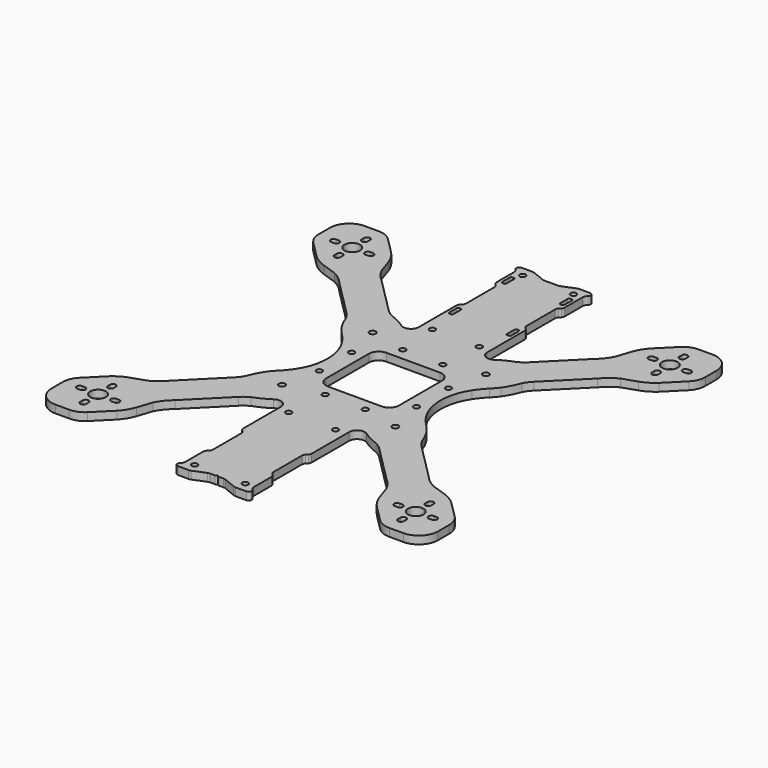
from build123d import *

# Parameters (mm, degrees)
F0_R     = 4
F0_R_2   = 1.5
F0_R_3   = 1.6
F1_DEPTH = 4


# Not quite as in the source:
# - ends of sketch curves that miss each other by under 0.0002 mm in the source are joined


with BuildPart() as f1:
    # F0 (on Top) → F1 (new body)
    with BuildSketch(Plane.XY):
        with BuildLine():
            ThreePointArc((-68.7198979633, -19.2310683136), (-69.2667474289, -19.0706292261), (-69.8340699923, -19.0164983863))
            Line((-69.8340699923, -19.0164983863), (-75.2563229923, -19.0164983863))
            ThreePointArc((-75.2563229923, -19.0164983863), (-76.6575815321, -19.9812652551), (-76.2563229867, -21.63453238))
            ThreePointArc((-76.2563229867, -21.63453238), (-75.5177102079, -22.645855508), (-75.2563229923, -23.8706003863))
            Line((-75.2563229923, -23.8706003863), (-75.2563229923, -35.1880713863))
            ThreePointArc((-75.2563229923, -35.1880713863), (-75.1040821926, -35.9534379244), (-74.6705370547, -36.6022844487))
            Line((-74.6705370547, -36.6022844487), (-73.8421089923, -37.4307123863))
            ThreePointArc((-73.8421089923, -37.4307123863), (-73.408563792, -38.0795588482), (-73.2563229923, -38.8449253863))
            Line((-73.2563229923, -38.8449253863), (-73.2563229923, -57.1880713863))
            ThreePointArc((-73.2563229923, -57.1880713863), (-73.408563792, -57.9534379244), (-73.8421089299, -58.6022844487))
            Line((-73.8421089299, -58.6022844487), (-74.6705369923, -59.4307123863))
            ThreePointArc((-74.6705369923, -59.4307123863), (-75.1040821926, -60.0795588482), (-75.2563229923, -60.8449253863))
            Line((-75.2563229923, -60.8449253863), (-75.2563229923, -84.8364823863))
            ThreePointArc((-75.2563229923, -84.8364823863), (-77.3940816238, -88.3765469458), (-81.5223515351, -88.1327097212))
            ThreePointArc((-81.5223515351, -88.1327097212), (-85.5001057777, -85.7657105269), (-89.7529047165, -83.9384406075))
            ThreePointArc((-89.7529047165, -83.9384406075), (-91.8824323761, -82.6525966161), (-93.7563230573, -81.0164984487))
            Line((-93.7563230573, -81.0164984487), (-111.8499919923, -62.9020143863))
            ThreePointArc((-111.8499919923, -62.9020143863), (-115.0500186095, -59.6637600428), (-117.5068461048, -55.8309464428))
            Line((-117.5068461048, -55.8309464428), (-119.9817199923, -48.4063253863))
            ThreePointArc((-119.9817199923, -48.4063253863), (-121.7314401326, -44.6478315667), (-124.2243601054, -41.3352574916))
            Line((-124.2243601054, -41.3352574916), (-132.7096419923, -32.8499763863))
            ThreePointArc((-132.7096419923, -32.8499763863), (-135.9638712469, -30.7325010032), (-139.7807099968, -30.0215490151))
            Line((-139.7807099968, -30.0215490151), (-146.8517769923, -30.0215493863))
            ThreePointArc((-146.8517769923, -30.0215493863), (-153.8517770371, -32.9210443415), (-156.7512719923, -39.9210443863))
            Line((-156.7512719923, -39.9210443863), (-156.7512719923, -46.9921113863))
            ThreePointArc((-156.7512719923, -46.9921113863), (-156.0403203754, -50.8089501317), (-153.9228453387, -54.0631797243))
            Line((-153.9228453387, -54.0631797243), (-145.4375639923, -62.5484613863))
            ThreePointArc((-145.4375639923, -62.5484613863), (-142.1249898119, -65.0413812461), (-138.3664962297, -66.7911020771))
            Line((-138.3664962297, -66.7911020771), (-130.9418749923, -69.2659753863))
            ThreePointArc((-130.9418749923, -69.2659753863), (-127.1090613358, -71.7228027691), (-123.870807081, -74.922829459))
            Line((-123.870807081, -74.922829459), (-105.8395839923, -92.9540523863))
            ThreePointArc((-105.8395839923, -92.9540523863), (-104.1591231129, -94.8555234649), (-102.8343796027, -97.0199161923))
            ThreePointArc((-102.8343796027, -97.0199161923), (-101.008160191, -101.2706562812), (-98.6427303315, -105.2466606194))
            ThreePointArc((-98.6427303315, -105.2466606194), (-97.1356962685, -107.0614279538), (-95.5198284171, -108.7800038111))
            ThreePointArc((-95.5198284171, -108.7800038111), (-93.1084062482, -111.4552655604), (-90.9867028572, -114.3656532981))
            ThreePointArc((-90.9867028572, -114.3656532981), (-86.6660489281, -129.0164983863), (-90.9867028572, -143.6673434744))
            ThreePointArc((-90.9867028572, -143.6673434744), (-93.1084062482, -146.5777312121), (-95.5198288752, -149.2529925034))
            ThreePointArc((-95.5198288752, -149.2529925034), (-97.1356962685, -150.9715688188), (-98.6427295666, -152.7863367182))
            ThreePointArc((-98.6427295666, -152.7863367182), (-101.008160191, -156.7623404914), (-102.8343807712, -161.0130801105))
            ThreePointArc((-102.8343807712, -161.0130801105), (-104.1591231129, -163.1774733076), (-105.8395836562, -165.0789447401))
            Line((-105.8395836562, -165.0789447401), (-123.8708069923, -183.1101673863))
            ThreePointArc((-123.8708069923, -183.1101673863), (-127.1090613358, -186.3101940035), (-130.9418749358, -188.7670214988))
            Line((-130.9418749358, -188.7670214988), (-138.3664959923, -191.2418953863))
            ThreePointArc((-138.3664959923, -191.2418953863), (-142.1249898119, -192.9916155265), (-145.437563887, -195.4845354993))
            Line((-145.437563887, -195.4845354993), (-153.9228449923, -203.9698173863))
            ThreePointArc((-153.9228449923, -203.9698173863), (-156.0403203754, -207.2240466409), (-156.7512723635, -211.0408853908))
            Line((-156.7512723635, -211.0408853908), (-156.7512719923, -218.1119523863))
            ThreePointArc((-156.7512719923, -218.1119523863), (-153.8517770371, -225.1119524311), (-146.8517769923, -228.0114473863))
            Line((-146.8517769923, -228.0114473863), (-139.7807099923, -228.0114473863))
            ThreePointArc((-139.7807099923, -228.0114473863), (-135.9638712469, -227.3004957694), (-132.7096416543, -225.1830207326))
            Line((-132.7096416543, -225.1830207326), (-124.2243599923, -216.6977393863))
            ThreePointArc((-124.2243599923, -216.6977393863), (-121.7314401326, -213.3851652059), (-119.9817193015, -209.6266716237))
            Line((-119.9817193015, -209.6266716237), (-117.5068459923, -202.2020503863))
            ThreePointArc((-117.5068459923, -202.2020503863), (-115.0500186095, -198.3692367297), (-111.8499919196, -195.130982475))
            Line((-111.8499919196, -195.130982475), (-93.7563229923, -177.0164983863))
            ThreePointArc((-93.7563229923, -177.0164983863), (-91.8824323761, -175.3804001564), (-89.7529048375, -174.0945557019))
            ThreePointArc((-89.7529048375, -174.0945557019), (-85.5001057777, -172.2672862456), (-81.5223513734, -169.9002872866))
            ThreePointArc((-81.5223513734, -169.9002872866), (-77.3940816238, -169.6564498268), (-75.2563229923, -173.1965143863))
            Line((-75.2563229923, -173.1965143863), (-75.2563229923, -197.1880713863))
            ThreePointArc((-75.2563229923, -197.1880713863), (-75.1040821926, -197.9534379244), (-74.6705370547, -198.6022844487))
            Line((-74.6705370547, -198.6022844487), (-73.8421089923, -199.4307123863))
            ThreePointArc((-73.8421089923, -199.4307123863), (-73.408563792, -200.0795588482), (-73.2563229923, -200.8449253863))
            Line((-73.2563229923, -200.8449253863), (-73.2563229923, -219.1880713863))
            ThreePointArc((-73.2563229923, -219.1880713863), (-73.408563792, -219.9534379244), (-73.8421089299, -220.6022844487))
            Line((-73.8421089299, -220.6022844487), (-74.6705369923, -221.4307123863))
            ThreePointArc((-74.6705369923, -221.4307123863), (-75.1040821926, -222.0795588482), (-75.2563229923, -222.8449253863))
            Line((-75.2563229923, -222.8449253863), (-75.2563229923, -234.1623963863))
            ThreePointArc((-75.2563229923, -234.1623963863), (-75.5177102079, -235.3871412645), (-76.2563230035, -236.3984643738))
            ThreePointArc((-76.2563230035, -236.3984643738), (-76.6575815321, -238.0517315174), (-75.2563229923, -239.0164983863))
            Line((-75.2563229923, -239.0164983863), (-69.8340699923, -239.0164983863))
            ThreePointArc((-69.8340699923, -239.0164983863), (-69.2667474289, -238.9623675465), (-68.7198979633, -238.8019284589))
            Line((-68.7198979633, -238.8019284589), (-62.2927479923, -236.2310683863))
            ThreePointArc((-62.2927479923, -236.2310683863), (-61.7458985558, -236.0706292261), (-61.1785759923, -236.0164983863))
            Line((-61.1785759923, -236.0164983863), (-58.7563229923, -236.0164983863))
            ThreePointArc((-58.7563229923, -236.0164983863), (-58.0492162111, -235.7236051675), (-57.7563229923, -235.0164983863))
            ThreePointArc((-57.7563229923, -235.0164983863), (-57.4634297735, -235.7236051675), (-56.7563229923, -236.0164983863))
            Line((-56.7563229923, -236.0164983863), (-54.3340699923, -236.0164983863))
            ThreePointArc((-54.3340699923, -236.0164983863), (-53.7667474289, -236.0706292261), (-53.2198979633, -236.2310683136))
            Line((-53.2198979633, -236.2310683136), (-46.7927479923, -238.8019283863))
            ThreePointArc((-46.7927479923, -238.8019283863), (-46.2458985558, -238.9623675465), (-45.6785759923, -239.0164983863))
            Line((-45.6785759923, -239.0164983863), (-40.2563229923, -239.0164983863))
            ThreePointArc((-40.2563229923, -239.0164983863), (-38.8550644525, -238.0517315174), (-39.2563229979, -236.3984643925))
            ThreePointArc((-39.2563229979, -236.3984643925), (-39.9949357768, -235.3871412645), (-40.2563229923, -234.1623963863))
            Line((-40.2563229923, -234.1623963863), (-40.2563229923, -222.8449253863))
            ThreePointArc((-40.2563229923, -222.8449253863), (-40.408563792, -222.0795588482), (-40.8421089299, -221.4307123239))
            Line((-40.8421089299, -221.4307123239), (-41.6705369923, -220.6022843863))
            ThreePointArc((-41.6705369923, -220.6022843863), (-42.1040821926, -219.9534379244), (-42.2563229923, -219.1880713863))
            Line((-42.2563229923, -219.1880713863), (-42.2563229923, -200.8449253863))
            ThreePointArc((-42.2563229923, -200.8449253863), (-42.1040821926, -200.0795588482), (-41.6705370547, -199.4307123239))
            Line((-41.6705370547, -199.4307123239), (-40.8421089923, -198.6022843863))
            ThreePointArc((-40.8421089923, -198.6022843863), (-40.408563792, -197.9534379244), (-40.2563229923, -197.1880713863))
            Line((-40.2563229923, -197.1880713863), (-40.2563229923, -173.1965143863))
            ThreePointArc((-40.2563229923, -173.1965143863), (-38.1185643608, -169.6564498268), (-33.9902944496, -169.9002870514))
            ThreePointArc((-33.9902944496, -169.9002870514), (-30.012540207, -172.2672862456), (-25.7597412681, -174.0945561651))
            ThreePointArc((-25.7597412681, -174.0945561651), (-23.6302136086, -175.3804001564), (-21.7563229274, -177.0164983238))
            Line((-21.7563229274, -177.0164983238), (-3.6626539923, -195.1309823863))
            ThreePointArc((-3.6626539923, -195.1309823863), (-0.4626273751, -198.3692367297), (1.9942001202, -202.2020503298))
            Line((1.9942001202, -202.2020503298), (4.4690740077, -209.6266713863))
            ThreePointArc((4.4690740077, -209.6266713863), (6.2187941479, -213.3851652059), (8.7117141207, -216.697739281))
            Line((8.7117141207, -216.697739281), (17.1969960077, -225.1830203863))
            ThreePointArc((17.1969960077, -225.1830203863), (20.4512252623, -227.3004957694), (24.2680640122, -228.0114477575))
            Line((24.2680640122, -228.0114477575), (31.3391310077, -228.0114473863))
            ThreePointArc((31.3391310077, -228.0114473863), (38.3391310525, -225.1119524311), (41.2386260077, -218.1119523863))
            Line((41.2386260077, -218.1119523863), (41.2386260077, -211.0408853863))
            ThreePointArc((41.2386260077, -211.0408853863), (40.5276743908, -207.2240466409), (38.410199354, -203.9698170483))
            Line((38.410199354, -203.9698170483), (29.9249180077, -195.4845353863))
            ThreePointArc((29.9249180077, -195.4845353863), (26.6123438273, -192.9916155265), (22.8538502451, -191.2418946955))
            Line((22.8538502451, -191.2418946955), (15.4292290077, -188.7670213863))
            ThreePointArc((15.4292290077, -188.7670213863), (11.5964153511, -186.3101940035), (8.3581610964, -183.1101673136))
            Line((8.3581610964, -183.1101673136), (-9.6730619923, -165.0789443863))
            ThreePointArc((-9.6730619923, -165.0789443863), (-11.3535228717, -163.1774733076), (-12.678266382, -161.0130805803))
            ThreePointArc((-12.678266382, -161.0130805803), (-14.5044857937, -156.7623404914), (-16.8699156531, -152.7863361531))
            ThreePointArc((-16.8699156531, -152.7863361531), (-18.3769497162, -150.9715688188), (-19.9928175675, -149.2529929615))
            ThreePointArc((-19.9928175675, -149.2529929615), (-22.4042397365, -146.5777312121), (-24.5259431274, -143.6673434744))
            ThreePointArc((-24.5259431274, -143.6673434744), (-28.8465970565, -129.0164983863), (-24.5259431274, -114.3656532981))
            ThreePointArc((-24.5259431274, -114.3656532981), (-22.4042397365, -111.4552655604), (-19.9928171095, -108.7800042691))
            ThreePointArc((-19.9928171095, -108.7800042691), (-18.3769497162, -107.0614279538), (-16.869916418, -105.2466600544))
            ThreePointArc((-16.869916418, -105.2466600544), (-14.5044857937, -101.2706562812), (-12.6782652135, -97.0199166621))
            ThreePointArc((-12.6782652135, -97.0199166621), (-11.3535228717, -94.8555234649), (-9.6730623284, -92.9540520325))
            Line((-9.6730623284, -92.9540520325), (8.3581610077, -74.9228293863))
            ThreePointArc((8.3581610077, -74.9228293863), (11.5964153511, -71.7228027691), (15.4292289512, -69.2659752738))
            Line((15.4292289512, -69.2659752738), (22.8538500077, -66.7911013863))
            ThreePointArc((22.8538500077, -66.7911013863), (26.6123438273, -65.0413812461), (29.9249179024, -62.5484612732))
            Line((29.9249179024, -62.5484612732), (38.4101990077, -54.0631793863))
            ThreePointArc((38.4101990077, -54.0631793863), (40.5276743908, -50.8089501317), (41.2386263789, -46.9921113818))
            Line((41.2386263789, -46.9921113818), (41.2386260077, -39.9210443863))
            ThreePointArc((41.2386260077, -39.9210443863), (38.3391310525, -32.9210443415), (31.3391310077, -30.0215493863))
            Line((31.3391310077, -30.0215493863), (24.2680640077, -30.0215493863))
            ThreePointArc((24.2680640077, -30.0215493863), (20.4512252623, -30.7325010032), (17.1969956697, -32.8499760399))
            Line((17.1969956697, -32.8499760399), (8.7117140077, -41.3352573863))
            ThreePointArc((8.7117140077, -41.3352573863), (6.2187941479, -44.6478315667), (4.4690733169, -48.4063251489))
            Line((4.4690733169, -48.4063251489), (1.9942000077, -55.8309463863))
            ThreePointArc((1.9942000077, -55.8309463863), (-0.4626273751, -59.6637600428), (-3.662654065, -62.9020142976))
            Line((-3.662654065, -62.9020142976), (-21.7563229923, -81.0164983863))
            ThreePointArc((-21.7563229923, -81.0164983863), (-23.6302136086, -82.6525966161), (-25.7597411471, -83.9384410707))
            ThreePointArc((-25.7597411471, -83.9384410707), (-30.012540207, -85.7657105269), (-33.9902946113, -88.1327094859))
            ThreePointArc((-33.9902946113, -88.1327094859), (-38.1185643608, -88.3765469458), (-40.2563229923, -84.8364823863))
            Line((-40.2563229923, -84.8364823863), (-40.2563229923, -60.8449253863))
            ThreePointArc((-40.2563229923, -60.8449253863), (-40.408563792, -60.0795588482), (-40.8421089299, -59.4307123239))
            Line((-40.8421089299, -59.4307123239), (-41.6705369923, -58.6022843863))
            ThreePointArc((-41.6705369923, -58.6022843863), (-42.1040821926, -57.9534379244), (-42.2563229923, -57.1880713863))
            Line((-42.2563229923, -57.1880713863), (-42.2563229923, -38.8449253863))
            ThreePointArc((-42.2563229923, -38.8449253863), (-42.1040821926, -38.0795588482), (-41.6705370547, -37.4307123239))
            Line((-41.6705370547, -37.4307123239), (-40.8421089923, -36.6022843863))
            ThreePointArc((-40.8421089923, -36.6022843863), (-40.408563792, -35.9534379244), (-40.2563229923, -35.1880713863))
            Line((-40.2563229923, -35.1880713863), (-40.2563229923, -23.8706003863))
            ThreePointArc((-40.2563229923, -23.8706003863), (-39.9949357768, -22.645855508), (-39.2563229811, -21.6345323988))
            ThreePointArc((-39.2563229811, -21.6345323988), (-38.8550644525, -19.9812652551), (-40.2563229923, -19.0164983863))
            Line((-40.2563229923, -19.0164983863), (-45.6785759923, -19.0164983863))
            ThreePointArc((-45.6785759923, -19.0164983863), (-46.2458985558, -19.0706292261), (-46.7927480214, -19.2310683136))
            Line((-46.7927480214, -19.2310683136), (-53.2198979923, -21.8019283863))
            ThreePointArc((-53.2198979923, -21.8019283863), (-53.7667474289, -21.9623675465), (-54.3340699923, -22.0164983863))
            Line((-54.3340699923, -22.0164983863), (-56.7563229923, -22.0164983863))
            Line((-56.7563229923, -22.0164983863), (-58.7563229923, -22.0164983863))
            Line((-58.7563229923, -22.0164983863), (-61.1785759923, -22.0164983863))
            ThreePointArc((-61.1785759923, -22.0164983863), (-61.7458985558, -21.9623675465), (-62.2927480214, -21.8019284589))
            Line((-62.2927480214, -21.8019284589), (-68.7198979633, -19.2310683136))
        make_face()
        with BuildLine():
            Line((-137.5736029923, -218.3337783863), (-137.5736029923, -219.8337783863))
            ThreePointArc((-137.5736029923, -219.8337783863), (-139.0736029923, -221.3337783863), (-140.5736029923, -219.8337783863))
            Line((-140.5736029923, -219.8337783863), (-140.5736029923, -218.3337783863))
            ThreePointArc((-140.5736029923, -218.3337783863), (-139.0736029923, -216.8337783863), (-137.5736029923, -218.3337783863))
        make_face(mode=Mode.SUBTRACT)
        with BuildLine():
            Line((-147.0736029923, -211.8337783863), (-148.5736029923, -211.8337783863))
            ThreePointArc((-148.5736029923, -211.8337783863), (-150.0736029923, -210.3337783863), (-148.5736029923, -208.8337783863))
            Line((-148.5736029923, -208.8337783863), (-147.0736029923, -208.8337783863))
            ThreePointArc((-147.0736029923, -208.8337783863), (-145.5736029923, -210.3337783863), (-147.0736029923, -211.8337783863))
        make_face(mode=Mode.SUBTRACT)
        with Locations((-139.0736029923, -210.3337783863)):
            Circle(F0_R, mode=Mode.SUBTRACT)
        with BuildLine():
            Line((-137.5736029923, -200.8337783863), (-137.5736029923, -202.3337783863))
            ThreePointArc((-137.5736029923, -202.3337783863), (-139.0736029923, -203.8337783863), (-140.5736029923, -202.3337783863))
            Line((-140.5736029923, -202.3337783863), (-140.5736029923, -200.8337783863))
            ThreePointArc((-140.5736029923, -200.8337783863), (-139.0736029923, -199.3337783863), (-137.5736029923, -200.8337783863))
        make_face(mode=Mode.SUBTRACT)
        with BuildLine():
            ThreePointArc((-129.5736029923, -208.8337783863), (-128.0736029923, -210.3337783863), (-129.5736029923, -211.8337783863))
            Line((-129.5736029923, -211.8337783863), (-131.0736029923, -211.8337783863))
            ThreePointArc((-131.0736029923, -211.8337783863), (-132.5736029923, -210.3337783863), (-131.0736029923, -208.8337783863))
            Line((-131.0736029923, -208.8337783863), (-129.5736029923, -208.8337783863))
        make_face(mode=Mode.SUBTRACT)
        with Locations((-70.7563229923, -234.0164983863)):
            Circle(F0_R_2, mode=Mode.SUBTRACT)
        with Locations((-86.7563229923, -158.0164983863)):
            Circle(F0_R_3, mode=Mode.SUBTRACT)
        with Locations((-69.7563229923, -175.0164983863)):
            Circle(F0_R_2, mode=Mode.SUBTRACT)
        with Locations((-82.5810189923, -139.2982913863)):
            Circle(F0_R_2, mode=Mode.SUBTRACT)
        with Locations((-68.0390489923, -153.8402613863)):
            Circle(F0_R_2, mode=Mode.SUBTRACT)
        with Locations((-44.7563229923, -234.0164983863)):
            Circle(F0_R_2, mode=Mode.SUBTRACT)
        with BuildLine():
            ThreePointArc((25.0609570077, -219.8337783863), (23.5609570077, -221.3337783863), (22.0609570077, -219.8337783863))
            Line((22.0609570077, -219.8337783863), (22.0609570077, -218.3337783863))
            ThreePointArc((22.0609570077, -218.3337783863), (23.5609570077, -216.8337783863), (25.0609570077, -218.3337783863))
            Line((25.0609570077, -218.3337783863), (25.0609570077, -219.8337783863))
        make_face(mode=Mode.SUBTRACT)
        with BuildLine():
            ThreePointArc((14.0609570077, -211.8337783863), (12.5609570077, -210.3337783863), (14.0609570077, -208.8337783863))
            Line((14.0609570077, -208.8337783863), (15.5609570077, -208.8337783863))
            ThreePointArc((15.5609570077, -208.8337783863), (17.0609570077, -210.3337783863), (15.5609570077, -211.8337783863))
            Line((15.5609570077, -211.8337783863), (14.0609570077, -211.8337783863))
        make_face(mode=Mode.SUBTRACT)
        with Locations((23.5609570077, -210.3337783863)):
            Circle(F0_R, mode=Mode.SUBTRACT)
        with BuildLine():
            ThreePointArc((25.0609570077, -202.3337783863), (23.5609570077, -203.8337783863), (22.0609570077, -202.3337783863))
            Line((22.0609570077, -202.3337783863), (22.0609570077, -200.8337783863))
            ThreePointArc((22.0609570077, -200.8337783863), (23.5609570077, -199.3337783863), (25.0609570077, -200.8337783863))
            Line((25.0609570077, -200.8337783863), (25.0609570077, -202.3337783863))
        make_face(mode=Mode.SUBTRACT)
        with BuildLine():
            ThreePointArc((31.5609570077, -211.8337783863), (30.0609570077, -210.3337783863), (31.5609570077, -208.8337783863))
            Line((31.5609570077, -208.8337783863), (33.0609570077, -208.8337783863))
            ThreePointArc((33.0609570077, -208.8337783863), (34.5609570077, -210.3337783863), (33.0609570077, -211.8337783863))
            Line((33.0609570077, -211.8337783863), (31.5609570077, -211.8337783863))
        make_face(mode=Mode.SUBTRACT)
        with Locations((-45.7563229923, -175.0164983863)):
            Circle(F0_R_2, mode=Mode.SUBTRACT)
        with Locations((-28.7563229923, -158.0164983863)):
            Circle(F0_R_3, mode=Mode.SUBTRACT)
        with Locations((-47.4735969923, -153.8402613863)):
            Circle(F0_R_2, mode=Mode.SUBTRACT)
        with BuildLine():
            ThreePointArc((-76.4634297735, -115.3093916051), (-74.9989636794, -111.7738576992), (-71.4634297735, -110.3093916051))
            Line((-71.4634297735, -110.3093916051), (-44.0492162111, -110.3093916051))
            ThreePointArc((-44.0492162111, -110.3093916051), (-40.5136823052, -111.7738576992), (-39.0492162111, -115.3093916051))
            Line((-39.0492162111, -115.3093916051), (-39.0492162111, -142.7236051675))
            ThreePointArc((-39.0492162111, -142.7236051675), (-40.5136823052, -146.2591390734), (-44.0492162111, -147.7236051675))
            Line((-44.0492162111, -147.7236051675), (-71.4634297735, -147.7236051675))
            ThreePointArc((-71.4634297735, -147.7236051675), (-74.9989636794, -146.2591390734), (-76.4634297735, -142.7236051675))
            Line((-76.4634297735, -142.7236051675), (-76.4634297735, -115.3093916051))
        make_face(mode=Mode.SUBTRACT)
        with Locations((-32.9316269923, -139.2982913863)):
            Circle(F0_R_2, mode=Mode.SUBTRACT)
        with Locations((-82.5810189923, -118.7347053863)):
            Circle(F0_R_2, mode=Mode.SUBTRACT)
        with Locations((-68.0390489923, -104.1927353863)):
            Circle(F0_R_2, mode=Mode.SUBTRACT)
        with Locations((-86.7563229923, -100.0164983863)):
            Circle(F0_R_3, mode=Mode.SUBTRACT)
        with Locations((-69.7563229923, -83.0164983863)):
            Circle(F0_R_2, mode=Mode.SUBTRACT)
        with BuildLine():
            ThreePointArc((-148.5736029923, -49.1992183863), (-150.0736029923, -47.6992183863), (-148.5736029923, -46.1992183863))
            Line((-148.5736029923, -46.1992183863), (-147.0736029923, -46.1992183863))
            ThreePointArc((-147.0736029923, -46.1992183863), (-145.5736029923, -47.6992183863), (-147.0736029923, -49.1992183863))
            Line((-147.0736029923, -49.1992183863), (-148.5736029923, -49.1992183863))
        make_face(mode=Mode.SUBTRACT)
        with BuildLine():
            ThreePointArc((-140.5736029923, -55.6992183863), (-139.0736029923, -54.1992183863), (-137.5736029923, -55.6992183863))
            Line((-137.5736029923, -55.6992183863), (-137.5736029923, -57.1992183863))
            ThreePointArc((-137.5736029923, -57.1992183863), (-139.0736029923, -58.6992183863), (-140.5736029923, -57.1992183863))
            Line((-140.5736029923, -57.1992183863), (-140.5736029923, -55.6992183863))
        make_face(mode=Mode.SUBTRACT)
        with Locations((-139.0736029923, -47.6992183863)):
            Circle(F0_R, mode=Mode.SUBTRACT)
        with BuildLine():
            ThreePointArc((-131.0736029923, -49.1992183863), (-132.5736029923, -47.6992183863), (-131.0736029923, -46.1992183863))
            Line((-131.0736029923, -46.1992183863), (-129.5736029923, -46.1992183863))
            ThreePointArc((-129.5736029923, -46.1992183863), (-128.0736029923, -47.6992183863), (-129.5736029923, -49.1992183863))
            Line((-129.5736029923, -49.1992183863), (-131.0736029923, -49.1992183863))
        make_face(mode=Mode.SUBTRACT)
        with BuildLine():
            ThreePointArc((-140.5736029923, -38.1992183863), (-139.0736029923, -36.6992183863), (-137.5736029923, -38.1992183863))
            Line((-137.5736029923, -38.1992183863), (-137.5736029923, -39.6992183863))
            ThreePointArc((-137.5736029923, -39.6992183863), (-139.0736029923, -41.1992183863), (-140.5736029923, -39.6992183863))
            Line((-140.5736029923, -39.6992183863), (-140.5736029923, -38.1992183863))
        make_face(mode=Mode.SUBTRACT)
        with BuildLine():
            ThreePointArc((-73.6813229923, -62.6164983863), (-73.4616530782, -62.0861683004), (-72.9313229923, -61.8664983863))
            Line((-72.9313229923, -61.8664983863), (-72.2313229923, -61.8664983863))
            ThreePointArc((-72.2313229923, -61.8664983863), (-71.7009929064, -62.0861683004), (-71.4813229923, -62.6164983863))
            Line((-71.4813229923, -62.6164983863), (-71.4813229923, -67.4164983863))
            ThreePointArc((-71.4813229923, -67.4164983863), (-71.7009929064, -67.9468284722), (-72.2313229923, -68.1664983863))
            Line((-72.2313229923, -68.1664983863), (-72.9313229923, -68.1664983863))
            ThreePointArc((-72.9313229923, -68.1664983863), (-73.4616530782, -67.9468284722), (-73.6813229923, -67.4164983863))
            Line((-73.6813229923, -67.4164983863), (-73.6813229923, -62.6164983863))
        make_face(mode=Mode.SUBTRACT)
        with BuildLine():
            ThreePointArc((-73.6813229923, -28.6164983863), (-73.4616530782, -28.0861683004), (-72.9313229923, -27.8664983863))
            Line((-72.9313229923, -27.8664983863), (-72.2313229923, -27.8664983863))
            ThreePointArc((-72.2313229923, -27.8664983863), (-71.7009929064, -28.0861683004), (-71.4813229923, -28.6164983863))
            Line((-71.4813229923, -28.6164983863), (-71.4813229923, -33.4164983863))
            ThreePointArc((-71.4813229923, -33.4164983863), (-71.7009929064, -33.9468284722), (-72.2313229923, -34.1664983863))
            Line((-72.2313229923, -34.1664983863), (-72.9313229923, -34.1664983863))
            ThreePointArc((-72.9313229923, -34.1664983863), (-73.4616530782, -33.9468284722), (-73.6813229923, -33.4164983863))
            Line((-73.6813229923, -33.4164983863), (-73.6813229923, -28.6164983863))
        make_face(mode=Mode.SUBTRACT)
        with Locations((-70.7563229923, -24.0164983863)):
            Circle(F0_R_2, mode=Mode.SUBTRACT)
        with Locations((-47.4735969923, -104.1927353863)):
            Circle(F0_R_2, mode=Mode.SUBTRACT)
        with Locations((-32.9316269923, -118.7347053863)):
            Circle(F0_R_2, mode=Mode.SUBTRACT)
        with Locations((-45.7563229923, -83.0164983863)):
            Circle(F0_R_2, mode=Mode.SUBTRACT)
        with Locations((-28.7563229923, -100.0164983863)):
            Circle(F0_R_3, mode=Mode.SUBTRACT)
        with BuildLine():
            ThreePointArc((-41.8313229923, -67.4164983863), (-42.0509929064, -67.9468284722), (-42.5813229923, -68.1664983863))
            Line((-42.5813229923, -68.1664983863), (-43.2813229923, -68.1664983863))
            ThreePointArc((-43.2813229923, -68.1664983863), (-43.8116530782, -67.9468284722), (-44.0313229923, -67.4164983863))
            Line((-44.0313229923, -67.4164983863), (-44.0313229923, -62.6164983863))
            ThreePointArc((-44.0313229923, -62.6164983863), (-43.8116530782, -62.0861683004), (-43.2813229923, -61.8664983863))
            Line((-43.2813229923, -61.8664983863), (-42.5813229923, -61.8664983863))
            ThreePointArc((-42.5813229923, -61.8664983863), (-42.0509929064, -62.0861683004), (-41.8313229923, -62.6164983863))
            Line((-41.8313229923, -62.6164983863), (-41.8313229923, -67.4164983863))
        make_face(mode=Mode.SUBTRACT)
        with BuildLine():
            ThreePointArc((-41.8313229923, -33.4164983863), (-42.0509929064, -33.9468284722), (-42.5813229923, -34.1664983863))
            Line((-42.5813229923, -34.1664983863), (-43.2813229923, -34.1664983863))
            ThreePointArc((-43.2813229923, -34.1664983863), (-43.8116530782, -33.9468284722), (-44.0313229923, -33.4164983863))
            Line((-44.0313229923, -33.4164983863), (-44.0313229923, -28.6164983863))
            ThreePointArc((-44.0313229923, -28.6164983863), (-43.8116530782, -28.0861683004), (-43.2813229923, -27.8664983863))
            Line((-43.2813229923, -27.8664983863), (-42.5813229923, -27.8664983863))
            ThreePointArc((-42.5813229923, -27.8664983863), (-42.0509929064, -28.0861683004), (-41.8313229923, -28.6164983863))
            Line((-41.8313229923, -28.6164983863), (-41.8313229923, -33.4164983863))
        make_face(mode=Mode.SUBTRACT)
        with Locations((-44.7563229923, -24.0164983863)):
            Circle(F0_R_2, mode=Mode.SUBTRACT)
        with BuildLine():
            Line((15.5609570077, -49.1992183863), (14.0609570077, -49.1992183863))
            ThreePointArc((14.0609570077, -49.1992183863), (12.5609570077, -47.6992183863), (14.0609570077, -46.1992183863))
            Line((14.0609570077, -46.1992183863), (15.5609570077, -46.1992183863))
            ThreePointArc((15.5609570077, -46.1992183863), (17.0609570077, -47.6992183863), (15.5609570077, -49.1992183863))
        make_face(mode=Mode.SUBTRACT)
        with BuildLine():
            ThreePointArc((22.0609570077, -55.6992183863), (23.5609570077, -54.1992183863), (25.0609570077, -55.6992183863))
            Line((25.0609570077, -55.6992183863), (25.0609570077, -57.1992183863))
            ThreePointArc((25.0609570077, -57.1992183863), (23.5609570077, -58.6992183863), (22.0609570077, -57.1992183863))
            Line((22.0609570077, -57.1992183863), (22.0609570077, -55.6992183863))
        make_face(mode=Mode.SUBTRACT)
        with Locations((23.5609570077, -47.6992183863)):
            Circle(F0_R, mode=Mode.SUBTRACT)
        with BuildLine():
            Line((31.5609570077, -46.1992183863), (33.0609570077, -46.1992183863))
            ThreePointArc((33.0609570077, -46.1992183863), (34.5609570077, -47.6992183863), (33.0609570077, -49.1992183863))
            Line((33.0609570077, -49.1992183863), (31.5609570077, -49.1992183863))
            ThreePointArc((31.5609570077, -49.1992183863), (30.0609570077, -47.6992183863), (31.5609570077, -46.1992183863))
        make_face(mode=Mode.SUBTRACT)
        with BuildLine():
            Line((22.0609570077, -39.6992183863), (22.0609570077, -38.1992183863))
            ThreePointArc((22.0609570077, -38.1992183863), (23.5609570077, -36.6992183863), (25.0609570077, -38.1992183863))
            Line((25.0609570077, -38.1992183863), (25.0609570077, -39.6992183863))
            ThreePointArc((25.0609570077, -39.6992183863), (23.5609570077, -41.1992183863), (22.0609570077, -39.6992183863))
        make_face(mode=Mode.SUBTRACT)
    extrude(amount=F1_DEPTH)


solid = f1.part
